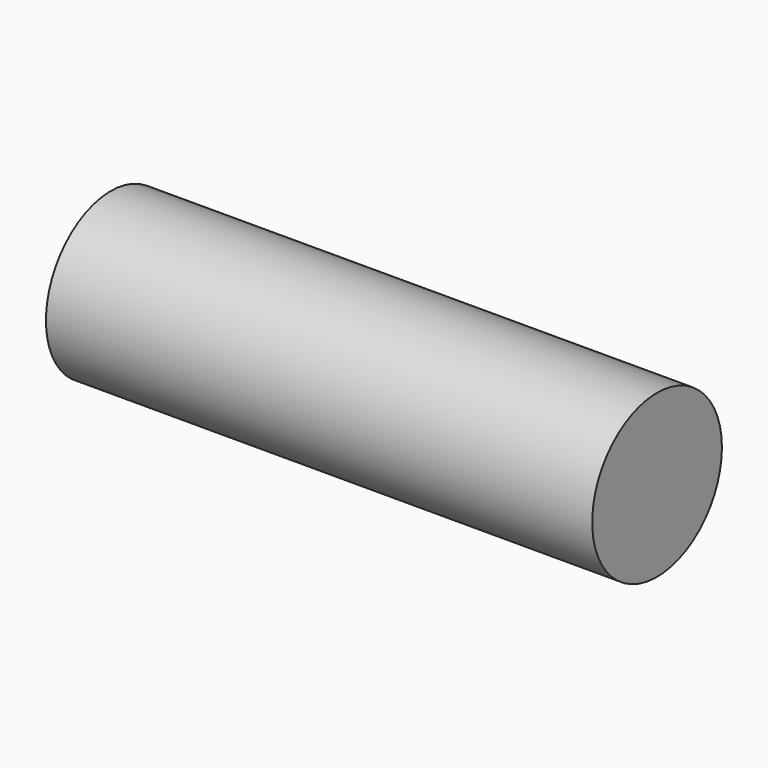
from build123d import *

# Parameters (mm, degrees)
F1_R     = 30.1625
F2_DEPTH = 101.6


# Not quite as in the source:
# - a variable given as a bare number and used for a length is read in inches; the dataset says mm whatever the document's units were


with BuildPart() as f2:
    # F1 (on Right) → F2 (new body, symmetric)
    with BuildSketch(Plane.YZ):
        Circle(F1_R)
    extrude(amount=F2_DEPTH, both=True)


solid = f2.part
